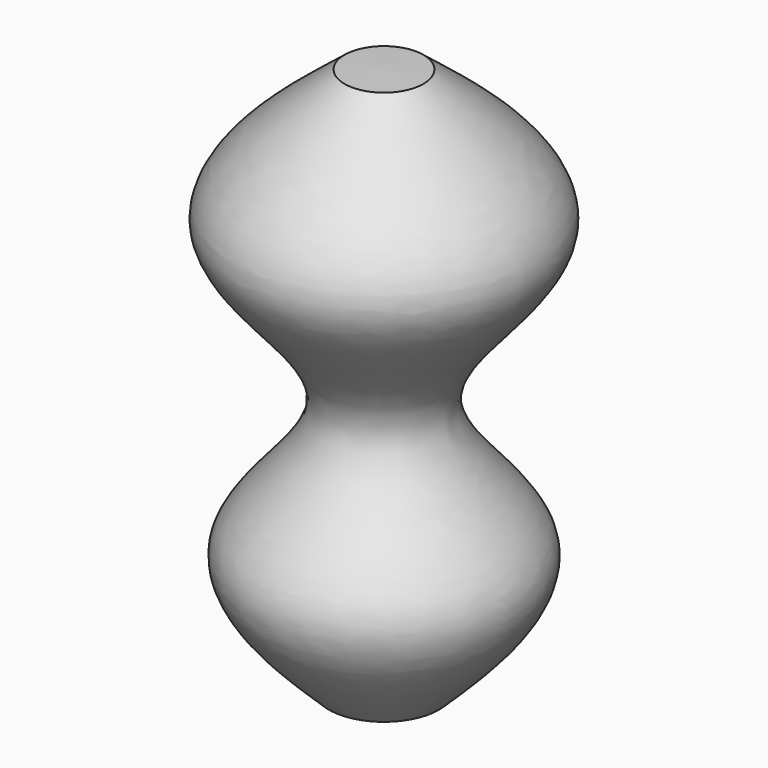
from build123d import *


# Not quite as in the source:
# - ends of sketch curves that miss each other by under 0.0002 mm in the source are joined
# - the dataset's text gives a spline's control points without its knots; the knots are read off the source's solid


with BuildPart() as f1:
    # F0 (on Front) → F1 (revolve)
    with BuildSketch(Plane.XZ):
        with BuildLine():
            Line((7.6182759816, 55.6974300589), (0, 55.8595135808))
            Line((0, 55.8595135808), (0, 52.4536972299))
            Line((0, 52.4536972299), (7.62, 52.4536972299))
            add(Edge.make_bspline(
                [(7.62, 52.4536972299), (8.4507741087, 51.7956075294), (10.6337911661, 50.0681673134), (14.0825299324, 47.2932496396), (17.7652011986, 44.139999809), (21.0139039479, 41.0293537983), (23.6727982156, 37.9850926484), (25.5952452636, 35.0543698089), (26.4978301822, 32.7719949731), (26.8001488213, 31.0502395533), (26.8193923693, 30.0008185238), (26.7295144932, 29.1588823674), (26.6074846335, 28.5247393458), (26.4233534744, 27.862329589), (26.0944531371, 26.9411497618), (25.528493763, 25.7246379164), (24.3188174109, 23.6687849146), (22.3143846414, 20.9480860054), (19.4254308568, 17.5470578663), (16.3687065974, 14.053414736), (13.9364574975, 11.0704228027), (12.2108797946, 8.6204173077), (11.0665218373, 6.7388599172), (10.1164243847, 4.7967330249), (9.5322697793, 3.1107263225), (9.2265726183, 1.714621277), (9.0889169388, 0.6460277237), (9.0559612523, -0.4446998408), (9.1305212863, -1.5148849791), (9.3003995532, -2.5611915369), (9.6403598774, -3.9195478282), (10.2508680098, -5.5467690428), (11.2076392915, -7.3988694604), (12.7073875743, -9.7620555753), (14.8851581339, -12.5648794621), (17.6572125501, -15.7773591275), (19.8337778082, -18.3521615832), (21.3317892611, -20.3374489686), (22.2940430686, -21.7788365909), (23.0586742875, -23.1572969124), (23.5990124042, -24.4555180702), (23.9006142985, -25.648512193), (24.0066287573, -26.8540972979), (23.9266033282, -28.0942726556), (23.5720177325, -29.8234035474), (22.655062987, -32.1412209964), (20.8358920917, -35.1217784732), (18.4115749368, -38.229977045), (15.5219332262, -41.4201740782), (12.312819371, -44.6646511445), (10.05718155, -46.8534319006), (8.9240978136, -47.9530082934)],
                knots=[0.0121327687, 0.0121327687, 0.0121327687, 0.0121327687, 0.03125, 0.0625, 0.09375, 0.125, 0.15625, 0.1875, 0.21875, 0.234375, 0.25, 0.2578125, 0.265625, 0.2734375, 0.28125, 0.296875, 0.3125, 0.34375, 0.375, 0.40625, 0.4375, 0.453125, 0.46875, 0.484375, 0.5, 0.5078125, 0.515625, 0.5234375, 0.53125, 0.5390625, 0.546875, 0.5625, 0.578125, 0.59375, 0.625, 0.65625, 0.6875, 0.703125, 0.71875, 0.734375, 0.75, 0.765625, 0.78125, 0.796875, 0.8125, 0.84375, 0.875, 0.90625, 0.9375, 0.96875, 1, 1, 1, 1], degree=3))
            Line((8.9240978136, -47.9530082934), (10.6929950416, -49.7758090496))
            add(Edge.make_bspline(
                [(7.6182759816, 55.6974300589), (19.0100411119, 46.6354798415), (42.9162754464, 29.0082902302), (-2.3090310079, 0.0342724215), (37.0155304225, -24.2479251585), (19.5054127389, -41.2239905455), (10.6929950416, -49.7758090496)],
                knots=[0, 0, 0, 0, 0.2631340266, 0.519760784, 0.7569409104, 1, 1, 1, 1], degree=3))
        make_face()
    revolve(axis=Axis((0, 0, 3.2262075692), (0, 0, -1)))


solid = f1.part
